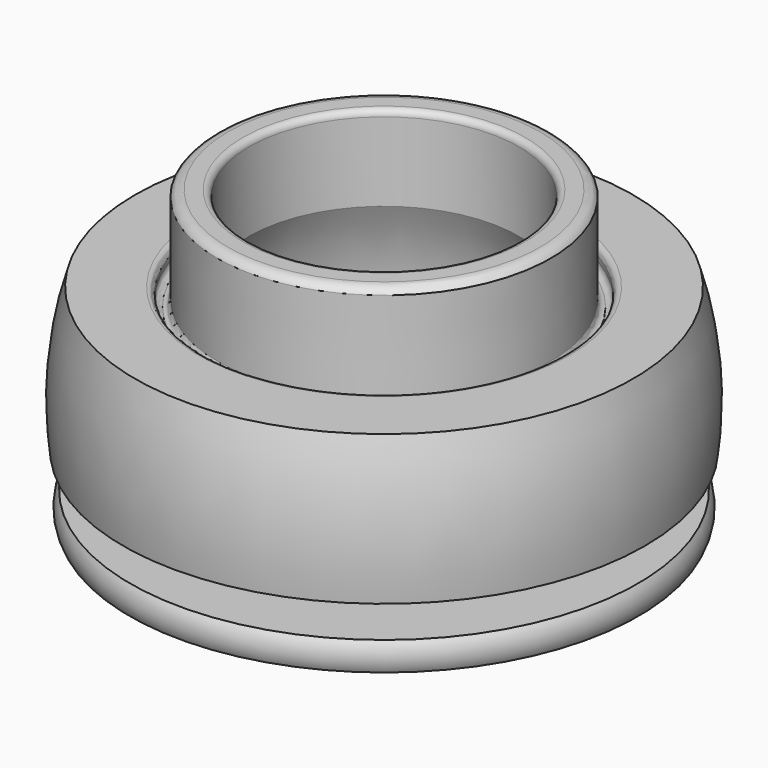
from build123d import *


# Not quite as in the source:
# - ends of sketch curves that miss each other by under 0.0002 mm in the source are joined
# - a feature names something its author has since deleted; it is built from what else it names


with BuildPart() as f1:
    # F0 (on Front) → F1 (revolve)
    with BuildSketch(Plane.XZ):
        with BuildLine():
            Line((-5.8782235887, 0.9034351679), (-8.0914394081, 0.9034351679))
            ThreePointArc((-8.0914394081, 0.9034351679), (-8.231987956, 0.4551696138), (-8.1157273695, 0))
            Line((-8.1157273695, 0), (-4.8928172328, 0))
            Line((-4.8928172328, 0), (-4.6930144623, 0.8424298139))
            ThreePointArc((-4.6930144623, 0.8424298139), (-5.0632580989, 3.778500016), (-4.2974063379, 6.63700656))
            Line((-4.2974063379, 6.63700656), (-4.2974063379, 9.1489921744))
            ThreePointArc((-4.2974063379, 9.1489921744), (-4.3559849816, 9.2904135306), (-4.4974063379, 9.3489921744))
            Line((-4.4974063379, 9.3489921744), (-4.9724063379, 9.3489921744))
            ThreePointArc((-4.9724063379, 9.3489921744), (-5.171105885, 9.2952208474), (-5.3155715691, 9.1485834315))
            Line((-5.3155715691, 9.1485834315), (-5.312120898, 6.2515290229))
            ThreePointArc((-5.312120898, 6.2515290229), (-5.3693549829, 6.1112267685), (-5.5085382742, 6.0513228918))
            Line((-5.5085382742, 6.0513228918), (-5.5121207562, 6.0512908038))
            ThreePointArc((-5.5121207562, 6.0512908038), (-5.6512200325, 6.1111417695), (-5.7085376994, 6.2512908038))
            Line((-5.7085376994, 6.2512908038), (-5.7085376994, 6.4135657753))
            ThreePointArc((-5.7085376994, 6.4135657753), (-5.7671163431, 6.5549871316), (-5.9085376994, 6.6135657753))
            Line((-5.9085376994, 6.6135657753), (-7.9404749973, 6.6135657753))
            ThreePointArc((-7.9404749973, 6.6135657753), (-8.3802520708, 4.3459608415), (-8.317330532, 2.0369617314))
            Line((-8.317330532, 2.0369617314), (-5.7418560656, 2.0369617314))
            ThreePointArc((-5.7418560656, 2.0369617314), (-5.3728936334, 1.4176081129), (-5.8782235887, 0.9034351679))
        make_face()
    revolve(axis=Axis((0.0153427809, 0, -114.6451877141), (0, 0, 1)))


with BuildPart() as f1_1:
    # F2: moved
    add(f1.part.moved(Location((0.025, 0, -0.1))))


solid = f1_1.part
